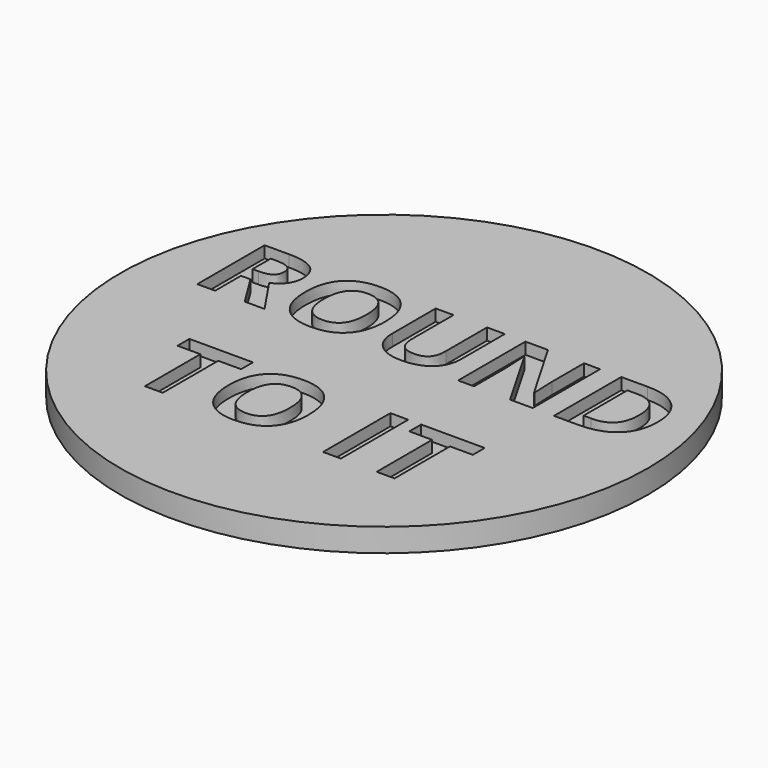
from build123d import *

# Parameters (mm, degrees)
F0_R         = 143.7377194923
F1_DEPTH     = 12.7
F2_TEXT_SIZE = 64.2032724702
F3_DEPTH     = 6.35


# Not quite as in the source:
# - Text() gives the source's letters only with a copy of the font that has no kerning and outlines rounded to 1/6400 em; it was checked with that copy


with BuildPart() as f1:
    # F0 (on Top) → F1 (new body)
    with BuildSketch(Plane.XY):
        Circle(F0_R)
    extrude(amount=F1_DEPTH)

    # F2 (on face) → F3 (cut)
    with BuildSketch(Plane.XY.offset(12.7)):
        with Locations((-117.6152378321, 12.656647712)):
            Text('ROUND', F2_TEXT_SIZE, font='Open Sans', font_style=FontStyle.BOLD, text_align=(TextAlign.LEFT, TextAlign.BOTTOM))
        with Locations((-84.2495996702, -74.6598028474)):
            Text('TO IT', F2_TEXT_SIZE, font='Open Sans', font_style=FontStyle.BOLD, text_align=(TextAlign.LEFT, TextAlign.BOTTOM))
    extrude(amount=-F3_DEPTH, mode=Mode.SUBTRACT)


solid = f1.part
